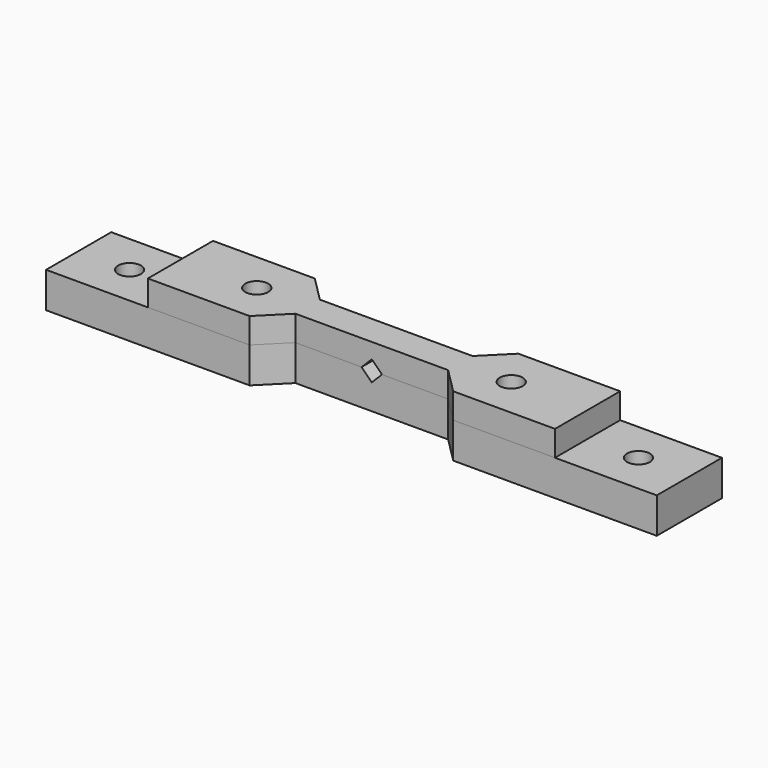
from build123d import *

# Parameters (mm, degrees)
F0_R     = 2.25
F1_DEPTH = 7
F3_DEPTH = 3
F4_DEPTH = 3
F5_R     = 2.25
F6_DEPTH = 5
F7_DEPTH = 5


with BuildPart() as f1:
    # F0 (on Top) → F1 (new body)
    with BuildSketch(Plane.XY):
        Polygon((0, -3), (0, 0), (0, 3), (-15, 3), (-20, 8), (-30, 8), (-54.389398545, 8), (-60, 8), (-60, -8), (-54.389398545, -8), (-30, -8), (-20, -8), (-15, -3), align=None)
        with Locations((-50, 0)):
            Circle(F0_R, mode=Mode.SUBTRACT)
        with Locations((-25, 0)):
            Circle(F0_R, mode=Mode.SUBTRACT)
        Polygon((0, 3), (0, 0), (0, -3), (15, -3), (20, -8), (30, -8), (53.1751337647, -8), (60, -8), (60, 8), (53.1751337647, 8), (30, 8), (20, 8), (15, 3), align=None)
        with Locations((25, 0)):
            Circle(F0_R, mode=Mode.SUBTRACT)
        with Locations((50, 0)):
            Circle(F0_R, mode=Mode.SUBTRACT)
    extrude(amount=F1_DEPTH)

    # F2 (on Front) → F3 (cut, symmetric)
    with BuildSketch(Plane.XZ):
        Polygon((2, 7), (-2, 7), (0, 5), align=None)
    extrude(amount=F3_DEPTH, both=True, mode=Mode.SUBTRACT)


with BuildPart() as f4:
    # F2 (on Front) → F4 (new body, symmetric)
    with BuildSketch(Plane.XZ):
        Polygon((-35, 7), (-15, 7), (-2, 7), (0, 9), (2, 7), (15, 7), (35, 7), (35, 12), (-35, 12), align=None)
    extrude(amount=F4_DEPTH, both=True)

    # F5 (on face) → F6 (join)
    with BuildSketch(Plane.XY.offset(7)):
        Polygon((-15, -3), (-15, 3), (-20, 8), (-40, 8), (-40, -8), (-20, -8), align=None)
        with Locations((-25, 0)):
            Circle(F5_R, mode=Mode.SUBTRACT)
        Polygon((20, 8), (15, 3), (15, -3), (20, -8), (40, -8), (40, 8), align=None)
        with Locations((25, 0)):
            Circle(F5_R, mode=Mode.SUBTRACT)
    extrude(amount=F6_DEPTH)

    # F5 (on face) → F7 (cut)
    with BuildSketch(Plane.XY.offset(7)):
        with Locations((-25, 0)):
            Circle(F5_R)
        with Locations((25, 0)):
            Circle(F5_R)
    extrude(amount=F7_DEPTH, mode=Mode.SUBTRACT)


solid = Compound([f1.part, f4.part])
